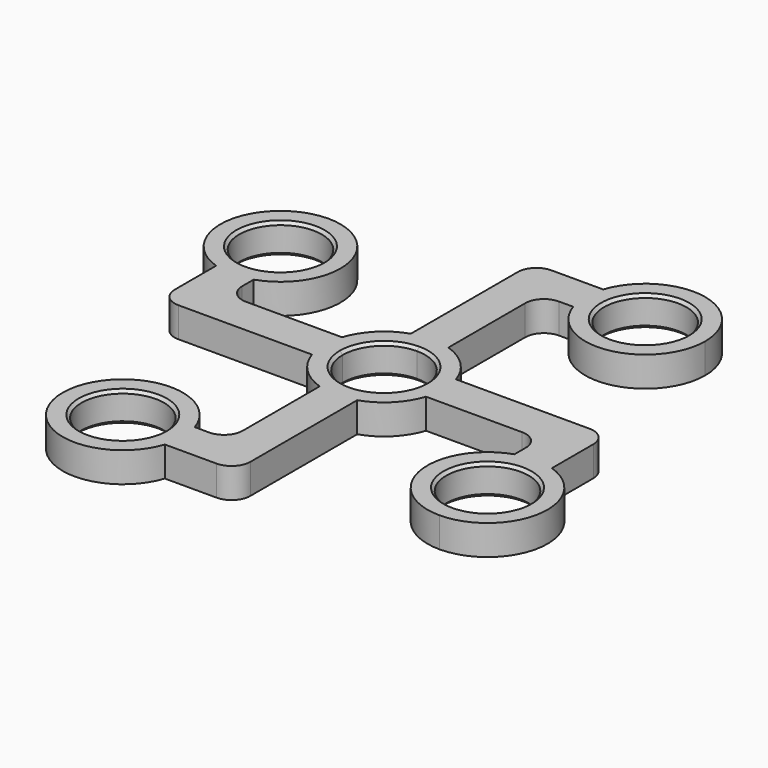
from build123d import *

# Parameters (mm, degrees)
F0_R     = 11
F1_DEPTH = 8
F3_COUNT = 4
F4_SIZE  = 0.762


# Not quite as in the source:
# - a feature names something its author has since deleted; it is built from what else it names


with BuildPart() as f1:
    # F0 (on Top) → F1 (new body)
    with BuildSketch(Plane.XY):
        with BuildLine():
            ThreePointArc((13.801315615, 55.7977184653), (13.2015990543, 53.3296207755), (13.0000001118, 50.7977195084))
            ThreePointArc((13.0000001118, 50.7977195084), (13.2015991411, 48.2658176992), (13.8013159582, 45.7977195084))
            ThreePointArc((13.8013159582, 45.7977195084), (31.531901921, 34.9993185378), (45.0000001118, 50.7977195084))
            ThreePointArc((45.0000001118, 50.7977195084), (31.5319013788, 66.5961205659), (13.801315615, 55.7977184653))
        make_face()
        with Locations((29.0000001118, 50.7977195084)):
            Circle(F0_R, mode=Mode.SUBTRACT)
        with BuildLine():
            Line((0, 50.7977195084), (0, 16))
            ThreePointArc((0, 16), (2.5319018092, 15.7984009706), (5, 15.1986841536))
            Line((5, 15.1986841536), (5, 40.7977195084))
            ThreePointArc((5, 40.7977195084), (6.4644660941, 44.3332534143), (10, 45.7977195084))
            Line((10, 45.7977195084), (13.8013159582, 45.7977195084))
            ThreePointArc((13.8013159582, 45.7977195084), (13.2015991411, 48.2658176992), (13.0000001118, 50.7977195084))
            Line((13.0000001118, 50.7977195084), (0, 50.7977195084))
        make_face()
        with BuildLine():
            ThreePointArc((-4.9999998882, 15.1986841903), (-2.5319017511, 15.7984009799), (0, 16))
            Line((0, 16), (0, 50.7977195084))
            Line((0, 50.7977195084), (13.0000001118, 50.7977195084))
            ThreePointArc((13.0000001118, 50.7977195084), (13.2015990543, 53.3296207755), (13.801315615, 55.7977184653))
            Line((13.801315615, 55.7977184653), (1.118e-07, 55.7977184653))
            ThreePointArc((1.118e-07, 55.7977184653), (-3.5355337942, 54.3332523713), (-4.9999998882, 50.7977184653))
            Line((-4.9999998882, 50.7977184653), (-4.9999998882, 15.1986841903))
        make_face()
        with BuildLine():
            ThreePointArc((5, 15.1986841536), (2.5319018092, 15.7984009706), (0, 16))
            ThreePointArc((0, 16), (-2.5319017511, 15.7984009799), (-4.9999998882, 15.1986841903))
            ThreePointArc((-4.9999998882, 15.1986841903), (-9.3808315673, -12.9614813623), (16, 0))
            ThreePointArc((16, 0), (12.9614813968, 9.3808315196), (5, 15.1986841536))
        make_face()
        with BuildLine():
            ThreePointArc((0, 11), (7.7781745931, 7.7781745931), (11, 0))
            ThreePointArc((11, 0), (-7.7781745931, -7.7781745931), (0, 11))
        make_face(mode=Mode.SUBTRACT)
    extrude(amount=F1_DEPTH)

    # F3: F1 ×4 about axis
    f3_axis = Axis((0, 0, 23.9773858339), (0, 0, 1))


with BuildPart() as f1_1:
    add(f1.part)
    for i in range(1, F3_COUNT):
        add(f1.part.rotate(f3_axis, i * 360 / F3_COUNT))

    # F4
    f4_edges = [f1_1.edges().sort_by_distance(p)[0] for p in [
        (-18, -50.79772, 8),
        (-50.79772, 18, 8),
        (18, 50.79772, 8),
        (50.79772, -18, 8),
        (0, -11, 8),
        (50.79772, -18, 0),
        (18, 50.79772, 0),
        (-50.79772, 18, 0),
        (0, -11, 0),
        (-18, -50.79772, 0),
    ]]
    chamfer(f4_edges, length=F4_SIZE)


solid = f1_1.part
